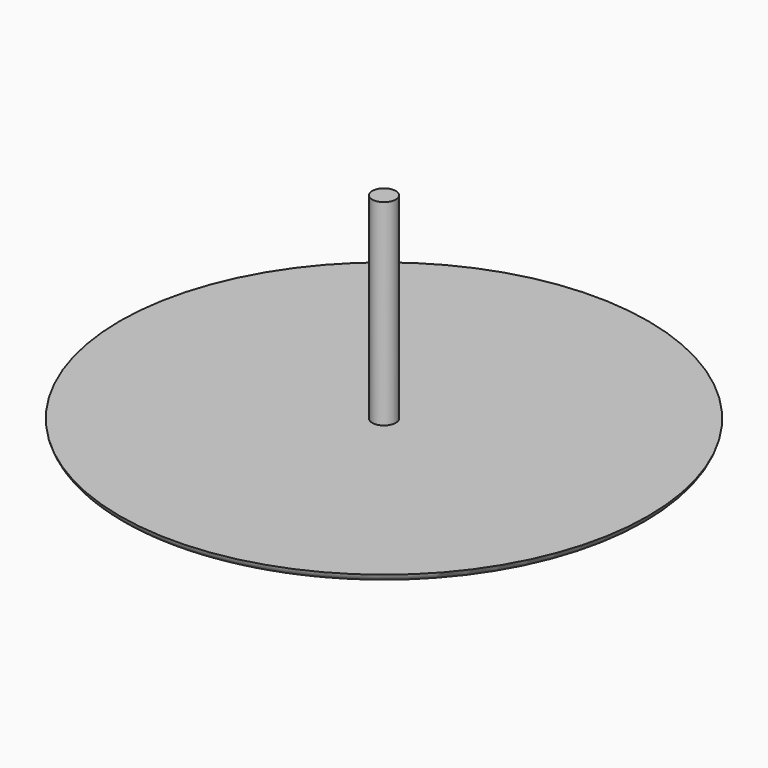
from build123d import *

# Parameters (mm, degrees)
F0_R     = 45
F0_R_2   = 2
F1_DEPTH = 1.5
F2_DEPTH = 35


# Not quite as in the source:
# - a fillet or chamfer that OpenCascade refuses, or shapes differently, is made with other operations: its cross-section is extruded or revolved along the edge and cut away or added


with BuildPart() as f1:
    # F0 (on Top) → F1 (new body)
    with BuildSketch(Plane.XY):
        Circle(F0_R)
        Circle(F0_R_2, mode=Mode.SUBTRACT)
    extrude(amount=F1_DEPTH)

    # F0 (on Top) → F2 (join)
    with BuildSketch(Plane.XY):
        Circle(F0_R_2)
    extrude(amount=F2_DEPTH)

    # F3: fillet of radius 2 on 1 edges, made by hand

    # F3_s1 → F3_t2 (revolve, cut)
    with BuildSketch(Plane.XZ):
        with BuildLine():
            ThreePointArc((45, 1.5), (44.2882531983, 0.4188611699), (43.0635083269, 0))
            Line((43.0635083269, 0), (45, 0))
            Line((45, 0), (45, 1.5))
        make_face()
    revolve(axis=Axis((0, 0, 0), (0, 0, 1)), mode=Mode.SUBTRACT)


solid = f1.part
